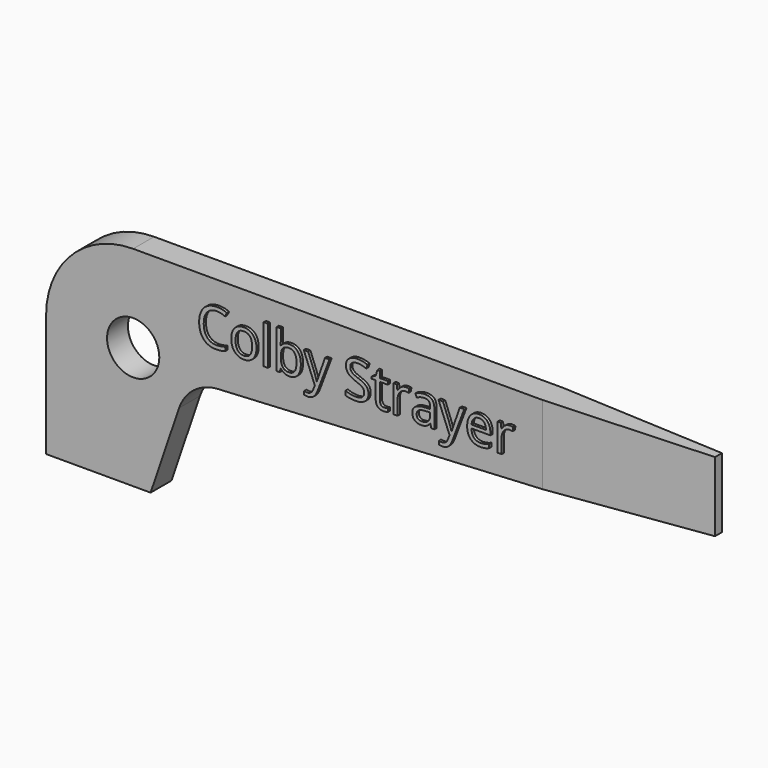
from build123d import *

# Parameters (mm, degrees)
F1_DEPTH     = 2.38125
F2_R         = 2.38125
F3_DEPTH     = 2.38225
F5_DEPTH     = 25.4
F6_TEXT_SIZE = 4.6700974269
F7_DEPTH     = 0.254


# Not quite as in the source:
# - Text() gives the source's letters only with a copy of the font that has no kerning and outlines rounded to 1/6400 em; it was checked with that copy


with BuildPart() as f1:
    # F0 (on Front) → F1 (new body)
    with BuildSketch(Plane.XZ):
        with BuildLine():
            Line((60.325, 19.05), (7.9375, 19.05))
            ThreePointArc((7.9375, 19.05), (2.3248399243, 16.7251600757), (0, 11.1125))
            Line((0, 11.1125), (0, 0))
            Line((0, 0), (9.525, 0))
            Line((9.525, 0), (12.1173647876, 7.6271664624))
            ThreePointArc((12.1173647876, 7.6271664624), (13.4786145605, 9.5135918491), (15.6631963617, 10.3130942181))
            Line((15.6631963617, 10.3130942181), (60.325, 12.7))
            Line((60.325, 12.7), (60.325, 19.05))
        make_face()
    extrude(amount=F1_DEPTH)

    # F2 (on face) → F3 (cut, through all)
    with BuildSketch(Plane.XZ.offset(2.38125)):
        with Locations((7.9375, 11.1125)):
            Circle(F2_R)
    extrude(amount=-F3_DEPTH, mode=Mode.SUBTRACT)

    # F4 (on face) → F5 (cut)
    with BuildSketch(Plane.XY.offset(19.05)):
        Polygon((60.325, 0), (45.24375, 0), (60.325, -0.79375), align=None)
        Polygon((60.325, -2.38125), (60.325, -1.5875), (45.24375, -2.38125), align=None)
    extrude(amount=-F5_DEPTH, mode=Mode.SUBTRACT)

    # F6 (on face) → F7 (join)
    with BuildSketch(Plane.XZ.offset(2.38125)):
        with Locations((13.8701874152, 13.6555298526)):
            Text('Colby Strayer', F6_TEXT_SIZE, font='Open Sans', text_align=(TextAlign.LEFT, TextAlign.BOTTOM))
    extrude(amount=F7_DEPTH)


solid = f1.part
